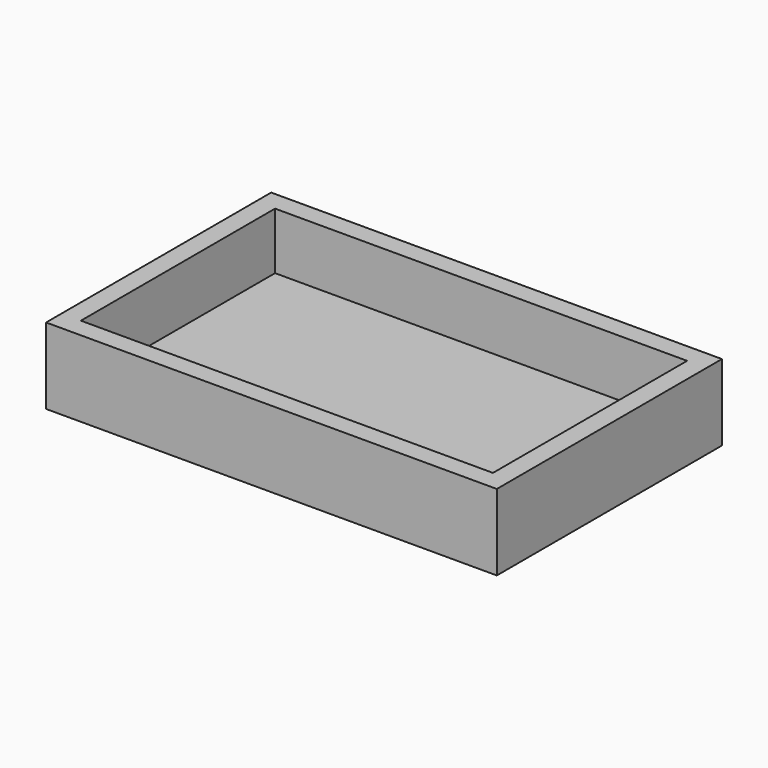
from build123d import *

# Parameters (mm, degrees)
F0_W     = 59.1892842203
F0_H     = 36.9495805353
F1_DEPTH = 10
F2_T     = -2.54


# Not quite as in the source:
# - the program builds the solid bodies; features that only make, move or delete a surface that nothing else refers to are left out


with BuildPart() as f1:
    # F0 (on Top) → F1 (new body)
    with BuildSketch(Plane.XY):
        with Locations((4.0522841737, -0.2056537196)):
            Rectangle(F0_W, F0_H)
    extrude(amount=F1_DEPTH)

    # F2
    f2_openings = [f1.faces().sort_by_distance(p)[0] for p in [
        (4.052284, -0.205654, 10),
    ]]
    offset(amount=F2_T, openings=f2_openings)


solid = f1.part
